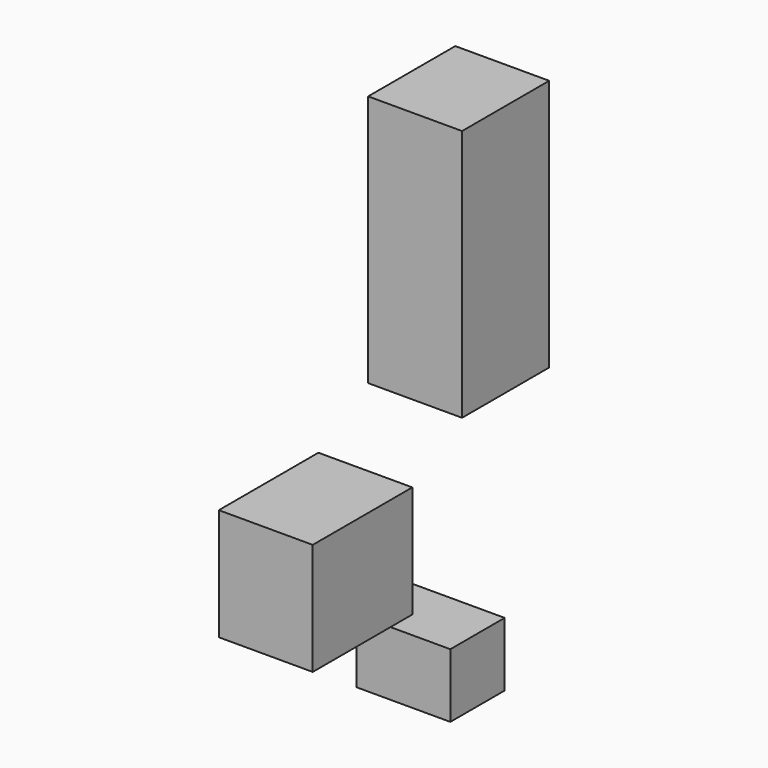
from build123d import *

# Parameters (mm, degrees)
F0_W     = 33.6623098701
F0_H     = 30.2589405328
F1_DEPTH = 25.4
F2_R     = 5.08
F3_T     = 2.54
F4_DEPTH = 25.4
F0_W_2   = 18.3612667024
F0_H_2   = 17.3079725355
F0_W_3   = 29.4476747513
F0_H_3   = 68.2704020292


# Not quite as in the source:
# - a shell that OpenCascade refuses in one call is made with other operations: the cavity is built on its own and cut out


with BuildPart() as f1:
    # F0 (on Right) → F1 (new body)
    with BuildSketch(Plane.YZ):
        with Locations((2.4481667206, 3.8996757939)):
            Rectangle(F0_W, F0_H)
    extrude(amount=F1_DEPTH)

    # F2
    f2_edges = [f1.edges().sort_by_distance(p)[0] for p in [
        (25.4, 2.448167, 19.029146),
        (25.4, -14.382988, 3.899676),
        (25.4, 2.448167, -11.229794),
        (25.4, 19.279322, 3.899676),
    ]]
    fillet(f2_edges, radius=F2_R)

    # F3: shell of thickness 2.54, made by hand


with BuildPart() as f3_core1:
    # F3_t2: copy of F1
    add(f1.part)

    # the walls: a layer under each face that stays
    f3_faces = [f3_core1.faces().sort_by_distance(p)[0] for p in [
        (10.16, 2.4481667206, 19.0291460603),
        (10.16, 19.2793216556, 3.8996757939),
        (23.9121024849, 2.4481667206, 17.5412484723),
        (23.9121024484, 17.7914241041, 3.8996757939),
        (23.9121024849, 2.4481667206, -9.7418968844),
    ]]
    thicken(f3_faces, amount=-F3_T, mode=Mode.SUBTRACT)


with BuildPart() as f1_1:
    add(f1.part)

    # what is left inside the walls is the cavity
    f3_cavity = [f3_core1.part.solids().sort_by_distance(p)[0] for p in [
        (0.0254, 1.178167, -1.990148),
    ]]
    add(f3_cavity, mode=Mode.SUBTRACT)

    # F0 (on Right) → F4 (join)
    with BuildSketch(Plane.YZ):
        with Locations((2.4481667206, 3.8996757939)):
            Rectangle(F0_W, F0_H)
    extrude(amount=F4_DEPTH)


with BuildPart() as f4:
    # F0 (on Right) → F4, piece 2 (new body)
    with BuildSketch(Plane.YZ):
        with Locations((41.3128491491, -33.3774806932)):
            Rectangle(F0_W_2, F0_H_2)
    extrude(amount=F4_DEPTH)


with BuildPart() as f4b:
    # F0 (on Right) → F4, piece 3 (new body)
    with BuildSketch(Plane.YZ):
        with Locations((50.818964839, 62.8925031051)):
            Rectangle(F0_W_3, F0_H_3)
    extrude(amount=F4_DEPTH)


solid = Compound([f1_1.part, f4.part, f4b.part])
